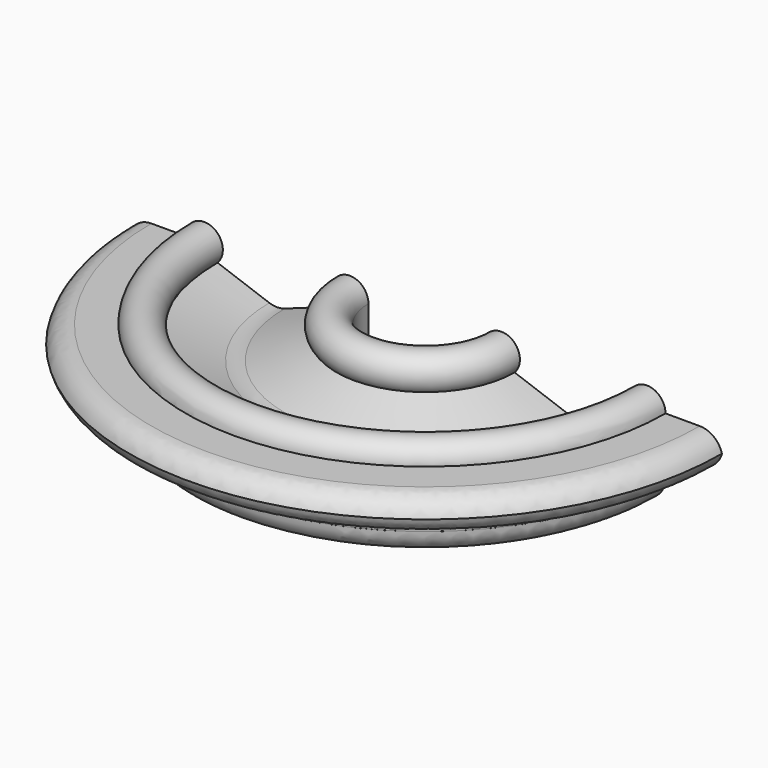
from build123d import *

# Parameters (mm, degrees)
F0_W        = 31.75
F0_H        = 19.05
F1_ANGLE    = 180
F2_R        = 12.7
F3_R        = 12.7
F4_T2_ANGLE = 202.072278
F4_T4_ANGLE = 202.072278
F4_T6_ANGLE = 207.327582


# Not quite as in the source:
# - a fillet or chamfer that OpenCascade refuses, or shapes differently, is made with other operations: its cross-section is extruded or revolved along the edge and cut away or added


with BuildPart() as f1:
    # F0 (on Front) → F1 (revolve)
    with BuildSketch(Plane.XZ):
        with Locations((-66.675, 22.225)):
            Rectangle(F0_W, F0_H)
        Polygon((50.8, -12.7), (50.8, 12.7), (0, 12.7), (-50.8, 12.7), (-50.8, -12.7), align=None)
        with BuildLine():
            Line((0, 12.7), (50.8, 12.7))
            Line((50.8, 12.7), (50.8, 31.75))
            ThreePointArc((50.8, 31.75), (36.564802, 41.32046), (33.074625, 24.52602))
            Line((33.074625, 24.52602), (0, 12.7))
        make_face()
        with BuildLine():
            Line((-50.8, 12.7), (0, 12.7))
            Line((0, 12.7), (-33.074625, 24.52602))
            ThreePointArc((-33.074625, 24.52602), (-36.564802, 41.32046), (-50.8, 31.75))
            Line((-50.8, 31.75), (-50.8, 12.7))
        make_face()
    revolve(axis=Axis((82.55, 0, 22.225), (0, 0, 1)), revolution_arc=F1_ANGLE)

    # F2
    f2_edges = [f1.edges().sort_by_distance(p)[0] for p in [
        (82.55, -82.55, 12.7),
    ]]
    fillet(f2_edges, radius=F2_R)

    # F3
    f3_edges = [f1.edges().sort_by_distance(p)[0] for p in [
        (82.55, -133.35, 12.7),
    ]]
    fillet(f3_edges, radius=F3_R)

    # F4: fillet of radius 12.7 on 3 edges, made by hand

    # F4_s1 → F4_t2 (revolve, cut)
    with BuildSketch(Plane(origin=(3.025022, 15.510151, 0), x_dir=(0, 0, 1), z_dir=(0.191428, 0.981507, 0))):
        with BuildLine():
            ThreePointArc((19.05, -84.076627), (28.030256, -80.356883), (31.75, -71.376627))
            Line((31.75, -71.376627), (31.75, -84.076627))
            Line((31.75, -84.076627), (19.05, -84.076627))
        make_face()
    revolve(axis=Axis((82.55, 0, 31.75), (0, 0, 1)), revolution_arc=F4_T2_ANGLE, mode=Mode.SUBTRACT)

    # F4_s3 → F4_t4 (revolve, cut)
    with BuildSketch(Plane(origin=(3.025022, 15.510151, 0), x_dir=(0, 0, 1), z_dir=(0.191428, 0.981507, 0))):
        with BuildLine():
            ThreePointArc((12.7, -71.376627), (16.419744, -80.356883), (25.4, -84.076627))
            Line((25.4, -84.076627), (12.7, -84.076627))
            Line((12.7, -84.076627), (12.7, -71.376627))
        make_face()
    revolve(axis=Axis((82.55, 0, 12.7), (0, 0, 1)), revolution_arc=F4_T4_ANGLE, mode=Mode.SUBTRACT)

    # F4_s5 → F4_t6 (revolve, cut)
    with BuildSketch(Plane(origin=(4.606441, 18.948415, 0), x_dir=(0, 0, 1), z_dir=(0.236224, 0.971699, 0))):
        with BuildLine():
            ThreePointArc((0, -53.136281), (-8.980256, -49.416537), (-12.7, -40.436281))
            Line((-12.7, -40.436281), (-12.7, -53.136281))
            Line((-12.7, -53.136281), (0, -53.136281))
        make_face()
    revolve(axis=Axis((82.55, 0, -12.7), (0, 0, 1)), revolution_arc=F4_T6_ANGLE, mode=Mode.SUBTRACT)


solid = f1.part
